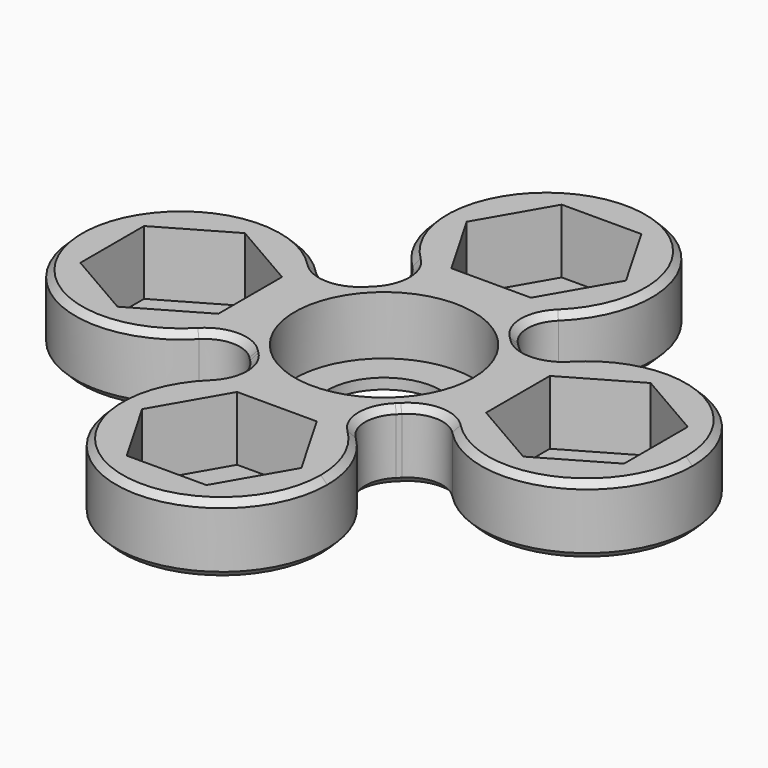
from build123d import *

# Parameters (mm, degrees)
F0_R     = 11
F0_R_2   = 7
F1_DEPTH = 0.6
F2_DEPTH = 8.5
F3_R     = 4.316991018
F4_SIZE  = 0.8
F5_DEPTH = 1.3


# Not quite as in the source:
# - a feature names something its author has since deleted; it is built from what else it names


with BuildPart() as f1:
    # F0 (on Top) → F1 (new body)
    with BuildSketch(Plane.XY):
        with BuildLine():
            ThreePointArc((-3.5707142143, 12.5), (0, 13), (3.5707142143, 12.5))
            ThreePointArc((3.5707142143, 12.5), (10.3783256064, 17.1711841504), (13, 25))
            ThreePointArc((13, 25), (-7.8288158496, 35.3783256064), (-3.5707142143, 12.5))
        make_face()
        Polygon((4.9074772881, 33.5), (9.8149545762, 25), (4.9074772881, 16.5), (-4.9074772881, 16.5), (-9.8149545762, 25), (-4.9074772881, 33.5), align=None, mode=Mode.SUBTRACT)
        with BuildLine():
            ThreePointArc((-12.5, -3.5707142143), (-13, 0), (-12.5, 3.5707142143))
            ThreePointArc((-12.5, 3.5707142143), (-38, 0), (-12.5, -3.5707142143))
        make_face()
        Polygon((-16.5, 4.9074772881), (-16.5, -4.9074772881), (-25, -9.8149545762), (-33.5, -4.9074772881), (-33.5, 4.9074772881), (-25, 9.8149545762), align=None, mode=Mode.SUBTRACT)
        with BuildLine():
            ThreePointArc((12.5, 3.5707142143), (12.8743931896, 1.8027756377), (13, 0))
            ThreePointArc((13, 0), (12.8743931896, -1.8027756377), (12.5, -3.5707142143))
            ThreePointArc((12.5, -3.5707142143), (26.8027756377, -12.8743931896), (38, 0))
            ThreePointArc((38, 0), (26.8027756377, 12.8743931896), (12.5, 3.5707142143))
        make_face()
        Polygon((16.5, -4.9074772881), (16.5, 4.9074772881), (25, 9.8149545762), (33.5, 4.9074772881), (33.5, -4.9074772881), (25, -9.8149545762), align=None, mode=Mode.SUBTRACT)
        with BuildLine():
            ThreePointArc((13, -25), (10.3783256064, -17.1711841504), (3.5707142143, -12.5))
            ThreePointArc((3.5707142143, -12.5), (0, -13), (-3.5707142143, -12.5))
            ThreePointArc((-3.5707142143, -12.5), (-7.8288158496, -35.3783256064), (13, -25))
        make_face()
        Polygon((-4.9074772881, -16.5), (4.9074772881, -16.5), (9.8149545762, -25), (4.9074772881, -33.5), (-4.9074772881, -33.5), (-9.8149545762, -25), align=None, mode=Mode.SUBTRACT)
        with BuildLine():
            ThreePointArc((12.5, -3.5707142143), (12, 0), (12.5, 3.5707142143))
            ThreePointArc((12.5, 3.5707142143), (9.1923881554, 9.1923881554), (3.5707142143, 12.5))
            ThreePointArc((3.5707142143, 12.5), (0, 12), (-3.5707142143, 12.5))
            ThreePointArc((-3.5707142143, 12.5), (-9.1923881554, 9.1923881554), (-12.5, 3.5707142143))
            ThreePointArc((-12.5, 3.5707142143), (-12.1256068104, 1.8027756377), (-12, 0))
            ThreePointArc((-12, 0), (-12.1256068104, -1.8027756377), (-12.5, -3.5707142143))
            ThreePointArc((-12.5, -3.5707142143), (-9.1923881554, -9.1923881554), (-3.5707142143, -12.5))
            ThreePointArc((-3.5707142143, -12.5), (0, -12), (3.5707142143, -12.5))
            ThreePointArc((3.5707142143, -12.5), (9.1923881554, -9.1923881554), (12.5, -3.5707142143))
        make_face()
        Circle(F0_R, mode=Mode.SUBTRACT)
        Circle(F0_R)
        Circle(F0_R_2, mode=Mode.SUBTRACT)
        Polygon((4.9074772881, 16.5), (9.8149545762, 25), (4.9074772881, 33.5), (-4.9074772881, 33.5), (-9.8149545762, 25), (-4.9074772881, 16.5), align=None)
        Polygon((-25, -9.8149545762), (-16.5, -4.9074772881), (-16.5, 4.9074772881), (-25, 9.8149545762), (-33.5, 4.9074772881), (-33.5, -4.9074772881), align=None)
        Polygon((25, 9.8149545762), (16.5, 4.9074772881), (16.5, -4.9074772881), (25, -9.8149545762), (33.5, -4.9074772881), (33.5, 4.9074772881), align=None)
        Polygon((9.8149545762, -25), (4.9074772881, -16.5), (-4.9074772881, -16.5), (-9.8149545762, -25), (-4.9074772881, -33.5), (4.9074772881, -33.5), align=None)
        with BuildLine():
            ThreePointArc((-3.5707142143, -12.5), (0, -13), (3.5707142143, -12.5))
            ThreePointArc((3.5707142143, -12.5), (0, -12), (-3.5707142143, -12.5))
        make_face()
        with BuildLine():
            ThreePointArc((12.5, -3.5707142143), (12.8743931896, -1.8027756377), (13, 0))
            ThreePointArc((13, 0), (12.8743931896, 1.8027756377), (12.5, 3.5707142143))
            ThreePointArc((12.5, 3.5707142143), (12, 0), (12.5, -3.5707142143))
        make_face()
        with BuildLine():
            ThreePointArc((-12, 0), (-12.1256068104, 1.8027756377), (-12.5, 3.5707142143))
            ThreePointArc((-12.5, 3.5707142143), (-13, 0), (-12.5, -3.5707142143))
            ThreePointArc((-12.5, -3.5707142143), (-12.1256068104, -1.8027756377), (-12, 0))
        make_face()
        with BuildLine():
            ThreePointArc((-3.5707142143, 12.5), (0, 12), (3.5707142143, 12.5))
            ThreePointArc((3.5707142143, 12.5), (0, 13), (-3.5707142143, 12.5))
        make_face()
    extrude(amount=F1_DEPTH)

    # F0 (on Top) → F2 (join)
    with BuildSketch(Plane.XY):
        with BuildLine():
            ThreePointArc((12.5, 3.5707142143), (12.8743931896, 1.8027756377), (13, 0))
            ThreePointArc((13, 0), (12.8743931896, -1.8027756377), (12.5, -3.5707142143))
            ThreePointArc((12.5, -3.5707142143), (26.8027756377, -12.8743931896), (38, 0))
            ThreePointArc((38, 0), (26.8027756377, 12.8743931896), (12.5, 3.5707142143))
        make_face()
        Polygon((16.5, -4.9074772881), (16.5, 4.9074772881), (25, 9.8149545762), (33.5, 4.9074772881), (33.5, -4.9074772881), (25, -9.8149545762), align=None, mode=Mode.SUBTRACT)
        with BuildLine():
            ThreePointArc((12.5, -3.5707142143), (12, 0), (12.5, 3.5707142143))
            ThreePointArc((12.5, 3.5707142143), (9.1923881554, 9.1923881554), (3.5707142143, 12.5))
            ThreePointArc((3.5707142143, 12.5), (0, 12), (-3.5707142143, 12.5))
            ThreePointArc((-3.5707142143, 12.5), (-9.1923881554, 9.1923881554), (-12.5, 3.5707142143))
            ThreePointArc((-12.5, 3.5707142143), (-12.1256068104, 1.8027756377), (-12, 0))
            ThreePointArc((-12, 0), (-12.1256068104, -1.8027756377), (-12.5, -3.5707142143))
            ThreePointArc((-12.5, -3.5707142143), (-9.1923881554, -9.1923881554), (-3.5707142143, -12.5))
            ThreePointArc((-3.5707142143, -12.5), (0, -12), (3.5707142143, -12.5))
            ThreePointArc((3.5707142143, -12.5), (9.1923881554, -9.1923881554), (12.5, -3.5707142143))
        make_face()
        Circle(F0_R, mode=Mode.SUBTRACT)
        with BuildLine():
            ThreePointArc((13, -25), (10.3783256064, -17.1711841504), (3.5707142143, -12.5))
            ThreePointArc((3.5707142143, -12.5), (0, -13), (-3.5707142143, -12.5))
            ThreePointArc((-3.5707142143, -12.5), (-7.8288158496, -35.3783256064), (13, -25))
        make_face()
        Polygon((-4.9074772881, -16.5), (4.9074772881, -16.5), (9.8149545762, -25), (4.9074772881, -33.5), (-4.9074772881, -33.5), (-9.8149545762, -25), align=None, mode=Mode.SUBTRACT)
        with BuildLine():
            ThreePointArc((-12.5, -3.5707142143), (-13, 0), (-12.5, 3.5707142143))
            ThreePointArc((-12.5, 3.5707142143), (-38, 0), (-12.5, -3.5707142143))
        make_face()
        Polygon((-16.5, 4.9074772881), (-16.5, -4.9074772881), (-25, -9.8149545762), (-33.5, -4.9074772881), (-33.5, 4.9074772881), (-25, 9.8149545762), align=None, mode=Mode.SUBTRACT)
        with BuildLine():
            ThreePointArc((-3.5707142143, 12.5), (0, 13), (3.5707142143, 12.5))
            ThreePointArc((3.5707142143, 12.5), (10.3783256064, 17.1711841504), (13, 25))
            ThreePointArc((13, 25), (-7.8288158496, 35.3783256064), (-3.5707142143, 12.5))
        make_face()
        Polygon((4.9074772881, 33.5), (9.8149545762, 25), (4.9074772881, 16.5), (-4.9074772881, 16.5), (-9.8149545762, 25), (-4.9074772881, 33.5), align=None, mode=Mode.SUBTRACT)
        with BuildLine():
            ThreePointArc((12.5, -3.5707142143), (12.8743931896, -1.8027756377), (13, 0))
            ThreePointArc((13, 0), (12.8743931896, 1.8027756377), (12.5, 3.5707142143))
            ThreePointArc((12.5, 3.5707142143), (12, 0), (12.5, -3.5707142143))
        make_face()
        with BuildLine():
            ThreePointArc((-3.5707142143, -12.5), (0, -13), (3.5707142143, -12.5))
            ThreePointArc((3.5707142143, -12.5), (0, -12), (-3.5707142143, -12.5))
        make_face()
        with BuildLine():
            ThreePointArc((-12, 0), (-12.1256068104, 1.8027756377), (-12.5, 3.5707142143))
            ThreePointArc((-12.5, 3.5707142143), (-13, 0), (-12.5, -3.5707142143))
            ThreePointArc((-12.5, -3.5707142143), (-12.1256068104, -1.8027756377), (-12, 0))
        make_face()
        with BuildLine():
            ThreePointArc((-3.5707142143, 12.5), (0, 12), (3.5707142143, 12.5))
            ThreePointArc((3.5707142143, 12.5), (0, 13), (-3.5707142143, 12.5))
        make_face()
    extrude(amount=F2_DEPTH)

    # F3
    f3_edges = [f1.edges().sort_by_distance(p)[0] for p in [
        (-3.570714, 12.5, 4.25),
        (3.570714, 12.5, 4.25),
        (-12.5, -3.570714, 4.25),
        (-12.5, 3.570714, 4.25),
        (12.5, 3.570714, 4.25),
        (12.5, -3.570714, 4.25),
        (3.570714, -12.5, 4.25),
        (-3.570714, -12.5, 4.25),
    ]]
    fillet(f3_edges, radius=F3_R)

    # F4
    f4_edges = [f1.edges().sort_by_distance(p)[0] for p in [
        (-9.192388, 9.192388, 8.5),
        (-7.667506, 12.5, 8.5),
        (0, 38, 8.5),
        (7.667506, 12.5, 8.5),
        (9.192388, 9.192388, 8.5),
        (9.192388, 9.192388, 0),
        (7.667506, 12.5, 0),
        (0, 38, 0),
        (-7.667506, 12.5, 0),
        (-9.192388, 9.192388, 0),
        (38, 0, 8.5),
        (12.5, -7.667506, 8.5),
        (12.5, 7.667506, 8.5),
        (9.192388, -9.192388, 8.5),
        (7.667506, -12.5, 8.5),
        (0, -38, 8.5),
        (-7.667506, -12.5, 8.5),
        (-9.192388, -9.192388, 8.5),
        (-12.5, -7.667506, 8.5),
        (-12.5, 7.667506, 8.5),
        (-38, 0, 8.5),
        (12.5, 7.667506, 0),
        (-12.5, 7.667506, 0),
        (38, 0, 0),
        (-38, 0, 0),
        (12.5, -7.667506, 0),
        (-12.5, -7.667506, 0),
        (9.192388, -9.192388, 0),
        (-9.192388, -9.192388, 0),
        (7.667506, -12.5, 0),
        (-7.667506, -12.5, 0),
        (0, -38, 0),
    ]]
    chamfer(f4_edges, length=F4_SIZE)

    # F0 (on Top) → F5 (join)
    with BuildSketch(Plane.XY):
        Circle(F0_R)
        Circle(F0_R_2, mode=Mode.SUBTRACT)
    extrude(amount=F5_DEPTH)


solid = f1.part
